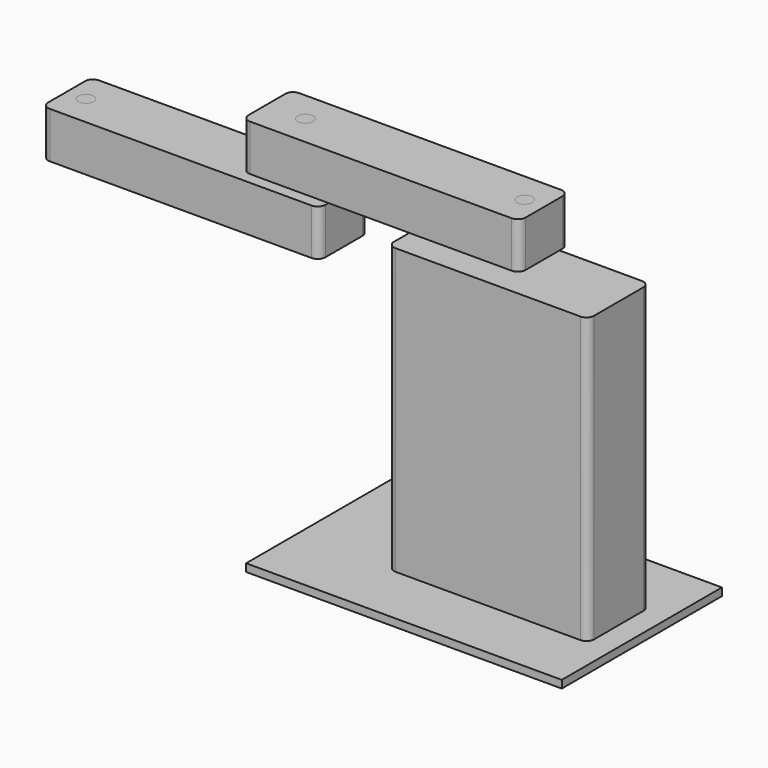
from build123d import *

# Parameters (mm, degrees)
F0_W      = 360
F0_H      = 80
F1_DEPTH  = 60
F3_W      = 260
F3_H      = 100
F4_DEPTH  = 370
F5_W      = 410
F5_H      = 260
F5_W_2    = 260
F5_H_2    = 100
F6_DEPTH  = 10
F7_W      = 360
F7_H      = 80
F8_DEPTH  = 60
F10_R     = 10
F10_2_R   = 10
F10_3_R   = 10
F11_T     = -4
F11_2_T   = -4
F11_3_T   = -4
F9_R      = 10
F12_DEPTH = 130
F13_DEPTH = 130
F14_R     = 10
F15_DEPTH = 60
F20_R     = 17.5
F20_R_2   = 10
F21_DEPTH = 10


# Not quite as in the source:
# - a feature names something its author has since deleted; it is built from what else it names


with BuildPart() as f1:
    # F0 (on Top) → F1 (new body)
    with BuildSketch(Plane.XY):
        Rectangle(F0_W, F0_H)
    extrude(amount=-F1_DEPTH)

    # F10
    f10_edges = [f1.edges().sort_by_distance(p)[0] for p in [
        (-180, -40, -30),
        (180, -40, -30),
        (180, 40, -30),
        (-180, 40, -30),
    ]]
    fillet(f10_edges, radius=F10_R)

    # F11
    f11_openings = [f1.faces().sort_by_distance(p)[0] for p in [
        (0, 0, -60),
    ]]
    offset(amount=F11_T, openings=f11_openings)


with BuildPart() as f4:
    # F3 (on offset) → F4 (new body)
    with BuildSketch(Plane.XY.offset(-70)):
        with Locations((155, -10)):
            Rectangle(F3_W, F3_H)
    extrude(amount=-F4_DEPTH)

    # F10#2
    f10_2_edges = [f4.edges().sort_by_distance(p)[0] for p in [
        (25, 40, -255),
        (25, -60, -255),
        (285, 40, -255),
        (285, -60, -255),
    ]]
    fillet(f10_2_edges, radius=F10_2_R)

    # F11#3
    f11_3_openings = [f4.faces().sort_by_distance(p)[0] for p in [
        (155, -10, -440),
    ]]
    offset(amount=F11_3_T, openings=f11_3_openings)


with BuildPart() as f6:
    # F5 (on face) → F6 (new body)
    with BuildSketch(Plane(origin=(0, 0, -440), x_dir=(1, 0, 0), z_dir=(0, 0, -1))):
        with Locations((110, 10)):
            Rectangle(F5_W, F5_H)
        with Locations((155, 10)):
            Rectangle(F5_W_2, F5_H_2, mode=Mode.SUBTRACT)
        with Locations((155, 10)):
            Rectangle(F5_W_2, F5_H_2)
    extrude(amount=F6_DEPTH)


with BuildPart() as f8:
    # F7 (on face) → F8 (new body)
    with BuildSketch(Plane.XY.offset(-70)):
        with Locations((-260, 0)):
            Rectangle(F7_W, F7_H)
    extrude(amount=-F8_DEPTH)

    # F10#3
    f10_3_edges = [f8.edges().sort_by_distance(p)[0] for p in [
        (-440, -40, -100),
        (-440, 40, -100),
        (-80, 40, -100),
        (-80, -40, -100),
    ]]
    fillet(f10_3_edges, radius=F10_3_R)

    # F11#2
    f11_2_openings = [f8.faces().sort_by_distance(p)[0] for p in [
        (-260, 0, -130),
    ]]
    offset(amount=F11_2_T, openings=f11_2_openings)


with BuildPart() as f12_tool:
    # F9 (on face) → F12 (new body)
    with BuildSketch(Plane.XY):
        with Locations((-415, 0)):
            Circle(F9_R)
        with Locations((-130, 0)):
            Circle(F9_R)
        with Locations((155, 0)):
            Circle(F9_R)
    extrude(amount=-F12_DEPTH)


with BuildPart() as f1_1:
    add(f1.part)

    # F12: cut by f12_tool
    add(f12_tool.part, mode=Mode.SUBTRACT)


with BuildPart() as f4_1:
    add(f4.part)

    # F12: cut by f12_tool
    add(f12_tool.part, mode=Mode.SUBTRACT)


with BuildPart() as f8_1:
    add(f8.part)

    # F12: cut by f12_tool
    add(f12_tool.part, mode=Mode.SUBTRACT)


with BuildPart() as f13:
    # F9 (on face) → F13 (new body)
    with BuildSketch(Plane.XY):
        with Locations((-130, 0)):
            Circle(F9_R)
    extrude(amount=-F13_DEPTH)


with BuildPart() as f13b:
    # F9 (on face) → F13, piece 2 (new body)
    with BuildSketch(Plane.XY):
        with Locations((155, 0)):
            Circle(F9_R)
    extrude(amount=-F13_DEPTH)


with BuildPart() as f15:
    # F14 (on face) → F15 (new body)
    with BuildSketch(Plane.XY.offset(-70)):
        with Locations((-415, 0)):
            Circle(F14_R)
    extrude(amount=-F15_DEPTH)


with BuildPart() as f21:
    # F20 (on offset) → F21 (new body)
    with BuildSketch(Plane(origin=(0, 0, -107), x_dir=(1, 0, 0), z_dir=(0, 0, -1))):
        with Locations((-130, 0)):
            Circle(F20_R)
        with Locations((-130, 0)):
            Circle(F20_R_2, mode=Mode.SUBTRACT)
    extrude(amount=-F21_DEPTH)


solid = Compound([f6.part, f1_1.part, f4_1.part, f8_1.part, f13.part, f13b.part, f15.part])
